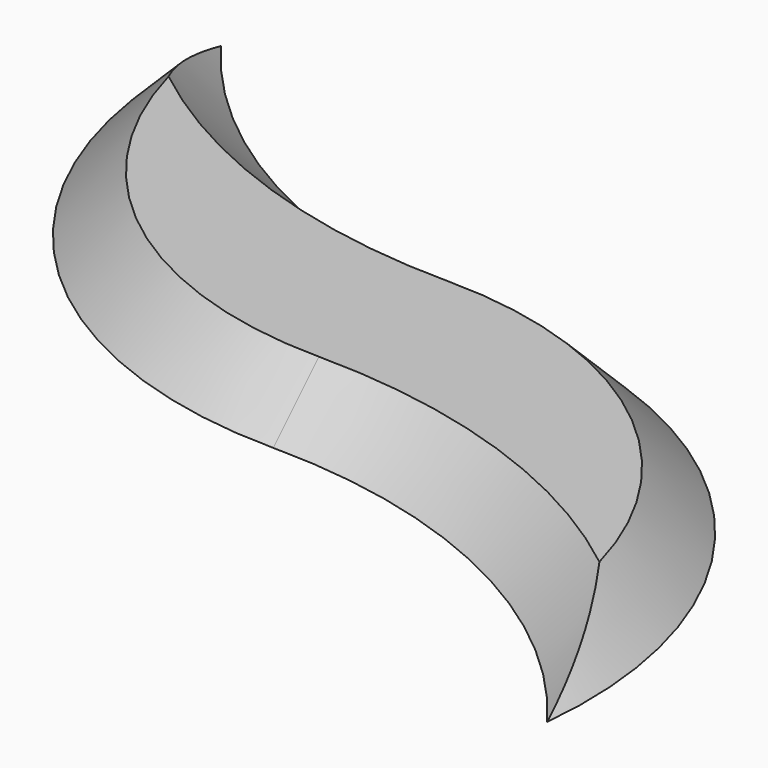
from build123d import *

# Parameters (mm, degrees)
F1_DEPTH = 2.5
F2_DEPTH = 2.5
F3_SIZE  = 2.49999


# Not quite as in the source:
# - a fillet or chamfer is up to 0.001 mm smaller than in the source, because OpenCascade refuses the exact size
# - a feature names something its author has since deleted; it is built from what else it names


with BuildPart() as f1:
    # F0 (on Top) → F1 (new body)
    with BuildSketch(Plane.XY):
        with BuildLine():
            ThreePointArc((-26.0619375711, 16.0619375711), (-20.9738946132, 0.5595870881), (-6.0619375711, -6.0619375711))
            Line((-6.0619375711, -6.0619375711), (-6.0619375711, 6.0619375711))
            ThreePointArc((-6.0619375711, 6.0619375711), (-17.2422774586, 8.7012577961), (-26.0619375711, 16.0619375711))
        make_face()
    extrude(amount=F1_DEPTH)

    # F0 (on Top) → F2 (join)
    with BuildSketch(Plane.XY):
        with BuildLine():
            Line((-6.0619375711, 6.0619375711), (-6.0619375711, -6.0619375711))
            ThreePointArc((-6.0619375711, -6.0619375711), (5.1184023164, -8.7012577961), (13.9380624289, -16.0619375711))
            ThreePointArc((13.9380624289, -16.0619375711), (8.8500194711, -0.5595870881), (-6.0619375711, 6.0619375711))
        make_face()
    extrude(amount=F2_DEPTH)

    # F3 (size 2.5 in the source; OpenCascade refuses exactly that, so slightly less here)
    f3_edges = [f1.edges().sort_by_distance(p)[0] for p in [
        (-20.973895, 0.559587, 2.5),
        (8.850019, -0.559587, 2.5),
    ]]
    chamfer(f3_edges, length=F3_SIZE)


solid = f1.part
